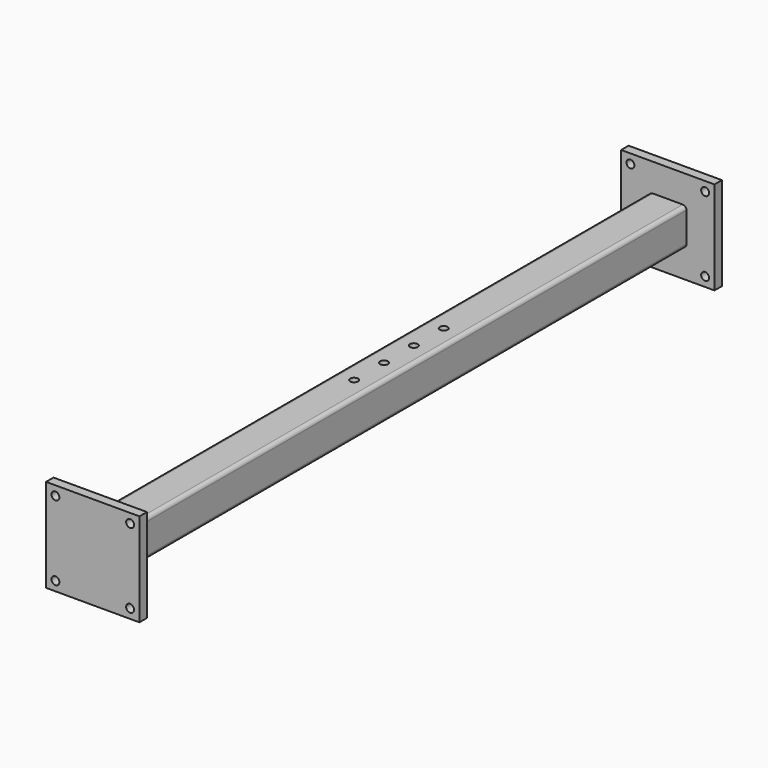
from build123d import *

# Parameters (mm, degrees)
F0_W           = 50.8
F0_H           = 50.8
F1_DEPTH       = 482.6
F2_W           = 127
F2_H           = 127
F2_W_2         = 50.8
F2_H_2         = 50.8
F3_DEPTH       = 12.7
F4_R           = 5.08
F5_D           = 10.71626
F9_D           = 10.71626
F9_DEPTH       = 31.2615384615
F9_TIP         = 3.2194893086
F9_ON_F8_D     = 10.71626
F9_ON_F8_DEPTH = 31.2615384615
F9_ON_F8_TIP   = 3.2194893086


# Not quite as in the source:
# - a feature names something its author has since deleted; it is built from what else it names


with BuildPart() as f1:
    # F0 (on Front) → F1 (new body, symmetric)
    with BuildSketch(Plane.XZ):
        Rectangle(F0_W, F0_H)
    extrude(amount=F1_DEPTH, both=True)

    # F2 (on face) → F3 (join)
    with BuildSketch(Plane.XZ.offset(482.6)):
        Rectangle(F2_W, F2_H)
        Rectangle(F2_W_2, F2_H_2, mode=Mode.SUBTRACT)
        Rectangle(F2_W_2, F2_H_2)
    extrude(amount=F3_DEPTH)

    # F4
    f4_edges = [f1.edges().sort_by_distance(p)[0] for p in [
        (25.4, 0, 25.4),
        (-25.4, 0, 25.4),
        (-25.4, 0, -25.4),
        (25.4, 0, -25.4),
    ]]
    fillet(f4_edges, radius=F4_R)

    # F5 (through all)
    with Locations(Plane(origin=(0, -482.6, 0), x_dir=(1, 0, 0), z_dir=(0, 1, 0))):
        with Locations((-50.8, -50.8), (50.8, -50.8), (50.8, 50.8), (-50.8, 50.8)):
            Hole(F5_D / 2)

    # F6: F1 across plane


with BuildPart() as f1_1:
    add(f1.part)
    add(f1.part.mirror(Plane.XZ))

    # F9
    with Locations(Plane(origin=(-25.4, 0, 0), x_dir=(0, -1, 0), z_dir=(-1, 0, 0))):
        with Locations((-50.8, 0), (50.8, 0), (-101.6, 0), (0, 0)):
            Hole(F9_D / 2, depth=F9_DEPTH)
            with Locations((0, 0, -(F9_DEPTH + F9_TIP / 2))):  # 118° drill point
                Cone(0, F9_D / 2, F9_TIP, mode=Mode.SUBTRACT)

    # F9 on F8
    with Locations(Plane.XY.offset(25.4)):
        with Locations((0, 0), (0, 101.6), (0, 50.8), (0, -50.8)):
            Hole(F9_ON_F8_D / 2, depth=F9_ON_F8_DEPTH)
            with Locations((0, 0, -(F9_ON_F8_DEPTH + F9_ON_F8_TIP / 2))):  # 118° drill point
                Cone(0, F9_ON_F8_D / 2, F9_ON_F8_TIP, mode=Mode.SUBTRACT)


solid = f1_1.part
